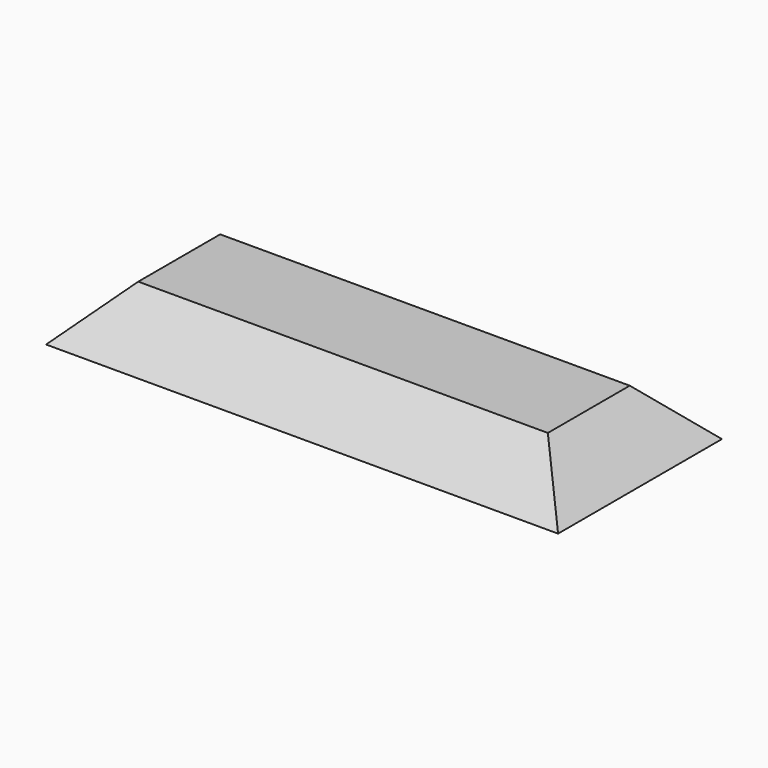
from build123d import *

# Parameters (mm, degrees)
F0_W     = 127
F0_H     = 12.7
F1_DEPTH = 25.4
F2_SIZE2 = 12.69999
F2_SIZE  = 12.69999


# Not quite as in the source:
# - a fillet or chamfer is up to 0.001 mm smaller than in the source, because OpenCascade refuses the exact size


with BuildPart() as f1:
    # F0 (on Front) → F1 (new body, symmetric)
    with BuildSketch(Plane.XZ):
        with Locations((0, 6.35)):
            Rectangle(F0_W, F0_H)
    extrude(amount=F1_DEPTH, both=True)

    # F2 (size 12.7 and 12.7 in the source; OpenCascade refuses exactly that, so slightly less here)
    f2_edges = [f1.edges().sort_by_distance(p)[0] for p in [
        (63.5, 0, 12.7),
        (0, 25.4, 12.7),
        (-63.5, 0, 12.7),
        (0, -25.4, 12.7),
    ]]
    chamfer(f2_edges, length=F2_SIZE, length2=F2_SIZE2)


solid = f1.part
